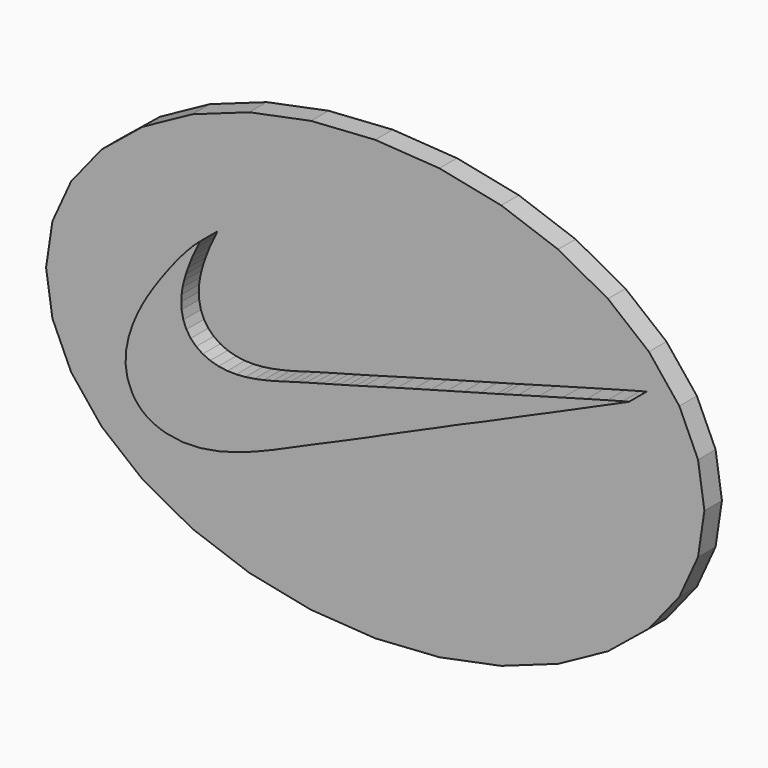
from build123d import *

# Parameters (mm, degrees)
F1_DEPTH = 3.175
F2_DEPTH = 6.35


# Not quite as in the source:
# - a length typed as a fraction of an inch, garbled in the dataset ("3 / 203.2 mm" for 3/8 in), is restored


with BuildPart() as f1:
    # F0 (on Front) → F1 (new body)
    with BuildSketch(Plane.XZ):
        Polygon((46.7098888, -6.1941202), (47.625, 0), (46.7098888, 6.1941202), (43.9997596, 12.150217), (39.598727, 17.6393602), (33.675955, 22.4506536), (26.4590276, 26.3991598), (18.2252874, 29.33319), (9.2911676, 31.1399428), (0, 31.75), (-9.291193, 31.1399428), (-18.2253128, 29.33319), (-26.459053, 26.3991598), (-33.6759804, 22.4506536), (-39.5987524, 17.6393602), (-43.999785, 12.150217), (-46.7099142, 6.1941202), (-47.625, 0), (-46.7099142, -6.1941202), (-43.999785, -12.1501916), (-39.5987524, -17.6393602), (-33.6759804, -22.4506282), (-26.459053, -26.3991598), (-18.2253128, -29.3331646), (-9.291193, -31.1399174), (0, -31.75), (9.2911676, -31.1399174), (18.2252874, -29.3331646), (26.4590276, -26.3991598), (33.675955, -22.4506282), (39.598727, -17.6393602), (43.9997596, -12.1501916), align=None)
        Polygon((38.341681, 12.2114056), (39.2552936, 12.4328174), (27.5334984, 7.2016112), (26.0539992, 6.5582038), (24.5790974, 5.9062112), (23.1074976, 5.2491132), (21.6381838, 4.590415), (20.1697844, 3.9334948), (18.7011818, 3.2820102), (17.2311822, 2.6391108), (15.7585918, 2.008505), (15.0165816, 1.6895064), (14.2783814, 1.3633196), (13.5421878, 1.0321036), (12.8065784, 0.6979158), (12.0698768, 0.362712), (11.3305844, 0.028702), (10.5870756, -0.3020822), (9.8377756, -0.6275832), (3.9710868, -3.244596), (2.5708864, -3.8890956), (1.1199876, -4.5439838), (-0.366014, -5.2049934), (-1.8718022, -5.8679842), (-3.38201, -6.5287906), (-4.8813212, -7.1831962), (-6.3541148, -7.8269846), (-7.7852016, -8.4560918), (-9.9900232, -9.4423992), (-12.3777248, -10.4928924), (-14.8971, -11.5218972), (-17.497425, -12.4434854), (-20.1276204, -13.1720844), (-22.7367084, -13.6216898), (-25.2738128, -13.706602), (-27.6880066, -13.341096), (-28.5486094, -13.0792982), (-29.3320216, -12.7701802), (-30.0423072, -12.4116846), (-30.6835048, -12.0018048), (-31.2595006, -11.5384834), (-31.774511, -11.0196884), (-32.2323206, -10.4433878), (-32.6370188, -9.8076004), (-33.312608, -8.1586832), (-33.575625, -6.422898), (-33.4963008, -4.6470824), (-33.1451204, -2.8779978), (-32.5923148, -1.1624818), (-31.9084198, 0.4526026), (-31.1636156, 1.9203162), (-30.4284126, 3.1938976), (-29.7318176, 4.2935144), (-28.9025076, 5.5216044), (-27.9718008, 6.8250054), (-26.9710154, 8.1507076), (-25.9315204, 9.4455996), (-24.8846086, 10.6565192), (-23.8617252, 11.7305074), (-22.8942138, 12.614402), (-22.9568248, 12.4025152), (-23.0575104, 12.1500138), (-23.185501, 11.8695978), (-23.3301032, 11.5739164), (-23.6254036, 10.9873034), (-23.857204, 10.491597), (-24.207724, 9.6268032), (-24.5462044, 8.744204), (-24.8575068, 7.8445106), (-25.1264166, 6.9283072), (-25.3376176, 5.9964066), (-25.4759206, 5.0494946), (-25.5260094, 4.0882062), (-25.4729234, 3.1132018), (-25.225121, 1.8998184), (-24.779605, 0.8263128), (-24.1524028, -0.1045972), (-23.3597196, -0.8900922), (-22.417405, -1.5274036), (-21.3416134, -2.0136866), (-20.1485246, -2.3462996), (-18.8540136, -2.5223978), (-17.5612044, -2.5464008), (-16.2439096, -2.449195), (-14.9162008, -2.2540976), (-13.591921, -1.9846036), (-12.2850148, -1.6639032), (-11.009503, -1.3152882), (-9.7794064, -0.9621012), (-8.6086188, -0.6277864), (-7.4149204, -0.2975864), (-6.2186058, 0.028702), (-5.0205132, 0.3525012), (-3.8219126, 0.6751066), (-2.6237184, 0.9980168), (-1.4270228, 1.3224002), (-0.2328164, 1.6497046), (0.9576816, 1.9814032), (3.358388, 2.652903), (5.7565798, 3.3170114), (8.152892, 3.9752016), (10.547985, 4.6289976), (12.942697, 5.2796186), (15.3375868, 5.928614), (17.7332894, 6.5773046), (20.1306938, 7.227316), (21.0277964, 7.4752962), (23.2002838, 8.0761078), (26.2238998, 8.910701), (29.6740834, 9.860407), (33.1267816, 10.806303), (36.1573826, 11.6296186), align=None, mode=Mode.SUBTRACT)
    extrude(amount=F1_DEPTH)

    # F0 (on Front) → F2 (join)
    with BuildSketch(Plane.XZ):
        Polygon((27.5334984, 7.2016112), (39.2552936, 12.4328174), (38.341681, 12.2114056), (36.1573826, 11.6296186), (33.1267816, 10.806303), (29.6740834, 9.860407), (26.2238998, 8.910701), (23.2002838, 8.0761078), (21.0277964, 7.4752962), (20.1306938, 7.227316), (17.7332894, 6.5773046), (15.3375868, 5.928614), (12.942697, 5.2796186), (10.547985, 4.6289976), (8.152892, 3.9752016), (5.7565798, 3.3170114), (3.358388, 2.652903), (0.9576816, 1.9814032), (-0.2328164, 1.6497046), (-1.4270228, 1.3224002), (-2.6237184, 0.9980168), (-3.8219126, 0.6751066), (-5.0205132, 0.3525012), (-6.2186058, 0.028702), (-7.4149204, -0.2975864), (-8.6086188, -0.6277864), (-9.7794064, -0.9621012), (-11.009503, -1.3152882), (-12.2850148, -1.6639032), (-13.591921, -1.9846036), (-14.9162008, -2.2540976), (-16.2439096, -2.449195), (-17.5612044, -2.5464008), (-18.8540136, -2.5223978), (-20.1485246, -2.3462996), (-21.3416134, -2.0136866), (-22.417405, -1.5274036), (-23.3597196, -0.8900922), (-24.1524028, -0.1045972), (-24.779605, 0.8263128), (-25.225121, 1.8998184), (-25.4729234, 3.1132018), (-25.5260094, 4.0882062), (-25.4759206, 5.0494946), (-25.3376176, 5.9964066), (-25.1264166, 6.9283072), (-24.8575068, 7.8445106), (-24.5462044, 8.744204), (-24.207724, 9.6268032), (-23.857204, 10.491597), (-23.6254036, 10.9873034), (-23.3301032, 11.5739164), (-23.185501, 11.8695978), (-23.0575104, 12.1500138), (-22.9568248, 12.4025152), (-22.8942138, 12.614402), (-23.8617252, 11.7305074), (-24.8846086, 10.6565192), (-25.9315204, 9.4455996), (-26.9710154, 8.1507076), (-27.9718008, 6.8250054), (-28.9025076, 5.5216044), (-29.7318176, 4.2935144), (-30.4284126, 3.1938976), (-31.1636156, 1.9203162), (-31.9084198, 0.4526026), (-32.5923148, -1.1624818), (-33.1451204, -2.8779978), (-33.4963008, -4.6470824), (-33.575625, -6.422898), (-33.312608, -8.1586832), (-32.6370188, -9.8076004), (-32.2323206, -10.4433878), (-31.774511, -11.0196884), (-31.2595006, -11.5384834), (-30.6835048, -12.0018048), (-30.0423072, -12.4116846), (-29.3320216, -12.7701802), (-28.5486094, -13.0792982), (-27.6880066, -13.341096), (-25.2738128, -13.706602), (-22.7367084, -13.6216898), (-20.1276204, -13.1720844), (-17.497425, -12.4434854), (-14.8971, -11.5218972), (-12.3777248, -10.4928924), (-9.9900232, -9.4423992), (-7.7852016, -8.4560918), (-6.3541148, -7.8269846), (-4.8813212, -7.1831962), (-3.38201, -6.5287906), (-1.8718022, -5.8679842), (-0.366014, -5.2049934), (1.1199876, -4.5439838), (2.5708864, -3.8890956), (3.9710868, -3.244596), (9.8377756, -0.6275832), (10.5870756, -0.3020822), (11.3305844, 0.028702), (12.0698768, 0.362712), (12.8065784, 0.6979158), (13.5421878, 1.0321036), (14.2783814, 1.3633196), (15.0165816, 1.6895064), (15.7585918, 2.008505), (17.2311822, 2.6391108), (18.7011818, 3.2820102), (20.1697844, 3.9334948), (21.6381838, 4.590415), (23.1074976, 5.2491132), (24.5790974, 5.9062112), (26.0539992, 6.5582038), align=None)
    extrude(amount=F2_DEPTH)


solid = f1.part
